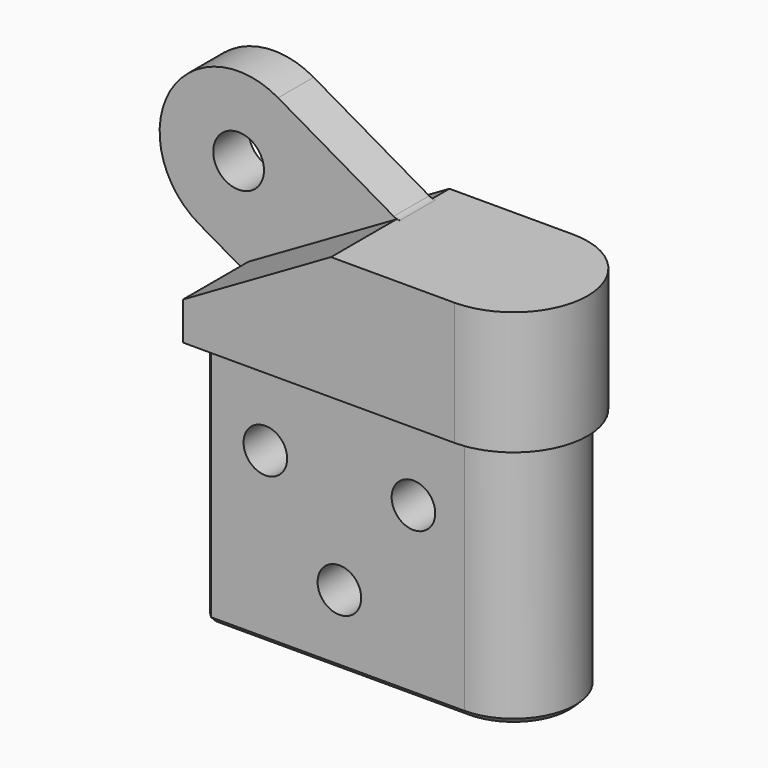
from build123d import *

# Parameters (mm, degrees)
F1_DEPTH = 15.875
F3_DEPTH = 31.75
F4_SIZE2 = 10.9985226281
F4_SIZE  = 19.05
F6_START = -2.794
F6_DEPTH = 5.715
F8_D     = 6.5278
F9_SIZE  = 0.762
F11_D    = 5.6134
F12_R    = 1.5875


with BuildPart() as f1:
    # F0 (on Top) → F1 (new body)
    with BuildSketch(Plane.XY):
        with BuildLine():
            Line((0, 9.525), (-34.925, 9.525))
            Line((-34.925, 9.525), (-34.925, -9.525))
            Line((-34.925, -9.525), (0, -9.525))
            ThreePointArc((0, -9.525), (9.525, 0), (0, 9.525))
        make_face()
    extrude(amount=-F1_DEPTH)

    # F2 (on face) → F3 (join)
    with BuildSketch(Plane(origin=(0, 0, -15.875), x_dir=(1, 0, 0), z_dir=(0, 0, -1))):
        with BuildLine():
            Line((0, 7.9375), (-33.3375, 7.9375))
            Line((-33.3375, 7.9375), (-33.3375, -7.9375))
            Line((-33.3375, -7.9375), (0, -7.9375))
            ThreePointArc((0, -7.9375), (7.9375, 0), (0, 7.9375))
        make_face()
    extrude(amount=F3_DEPTH)

    # F4
    f4_edges = [f1.edges().sort_by_distance(p)[0] for p in [
        (-34.925, 0, 0),
    ]]
    f4_side = f1.faces().sort_by_distance((-13.668751, 0, 0))[0]
    chamfer(f4_edges, length=F4_SIZE, length2=F4_SIZE2, reference=f4_side)

    # F5 (on face) → F6 (join)
    with BuildSketch(Plane(origin=(0, 9.525, 0), x_dir=(-1, 0, 0), z_dir=(0, 1, 0)).offset(F6_START)):
        with BuildLine():
            Line((34.925, -12.4649923118), (41.275, -8.7988181024))
            ThreePointArc((41.275, -8.7988181024), (44.9938181024, 5.08), (31.115, 8.7988181024))
            Line((31.115, 8.7988181024), (15.875, 0))
            Line((15.875, 0), (34.925, -10.9985226281))
            Line((34.925, -10.9985226281), (34.925, -12.4649923118))
        make_face()
    extrude(amount=-F6_DEPTH)

    # F8 (through all)
    with Locations(Plane(origin=(0, 6.731, 0), x_dir=(-1, 0, 0), z_dir=(0, 1, 0))):
        with Locations((36.195, 0)):
            Hole(F8_D / 2)

    # F9
    f9_edges = [f1.edges().sort_by_distance(p)[0] for p in [
        (-16.66875, -7.9375, -47.625),
        (-33.3375, 0, -47.625),
        (-33.3375, -7.9375, -31.75),
        (-33.3375, 7.9375, -31.75),
        (7.9375, 0, -47.625),
        (-16.66875, 7.9375, -47.625),
    ]]
    chamfer(f9_edges, length=F9_SIZE)

    # F11 (through all)
    with Locations(Plane(origin=(0, 7.9375, 0), x_dir=(-1, 0, 0), z_dir=(0, 1, 0))):
        with Locations((25.5905, -25.7175), (6.5405, -25.7175), (16.0655, -38.4175)):
            Hole(F11_D / 2)

    # F12
    f12_edges = [f1.edges().sort_by_distance(p)[0] for p in [
        (-15.875, 3.8735, 0),
        (-34.925, 3.8735, -12.464992),
    ]]
    fillet(f12_edges, radius=F12_R)


solid = f1.part
